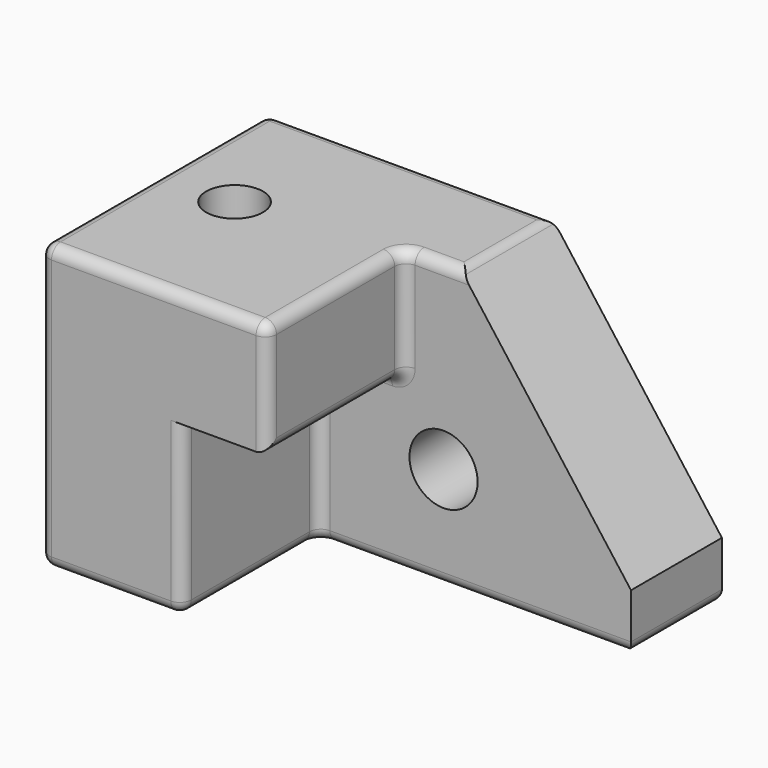
from build123d import *

# Parameters (mm, degrees)
F0_W     = 203.2
F0_H     = 127
F1_DEPTH = 127
F3_DEPTH = 76.2
F4_SIZE2 = 101.6
F4_SIZE  = 76.2
F5_R     = 5.08
F6_R     = 15.24
F7_DEPTH = 50.8
F8_R     = 12.7
F9_DEPTH = 127


with BuildPart() as f1:
    # F0 (on Front) → F1 (new body)
    with BuildSketch(Plane.XZ):
        Rectangle(F0_W, F0_H)
    extrude(amount=F1_DEPTH)

    # F2 (on face) → F3 (cut)
    with BuildSketch(Plane.XZ.offset(127)):
        Polygon((101.6, 63.5), (0, 63.5), (0, 12.7), (-38.1, 12.7), (-38.1, -63.5), (101.6, -63.5), align=None)
    extrude(amount=-F3_DEPTH, mode=Mode.SUBTRACT)

    # F4
    f4_edges = [f1.edges().sort_by_distance(p)[0] for p in [
        (101.6, -25.4, 63.5),
    ]]
    f4_side = f1.faces().sort_by_distance((-21.771429, -52.614286, 63.5))[0]
    chamfer(f4_edges, length=F4_SIZE, length2=F4_SIZE2, reference=f4_side)

    # F5
    f5_edges = [f1.edges().sort_by_distance(p)[0] for p in [
        (0, -88.9, 63.5),
        (12.7, -50.8, 63.5),
        (25.4, -25.4, 63.5),
        (-38.1, 0, 63.5),
        (-101.6, -63.5, 63.5),
        (-50.8, -127, 63.5),
        (0, -127, 38.1),
        (0, -88.9, 12.7),
        (0, -50.8, 38.1),
        (-38.1, -50.8, -25.4),
        (-38.1, -127, -25.4),
        (-38.1, -88.9, -63.5),
        (-69.85, -127, -63.5),
        (-101.6, -127, 0),
        (31.75, -50.8, -63.5),
        (101.6, -25.4, -63.5),
        (-101.6, -63.5, -63.5),
        (-101.6, 0, 0),
        (0, 0, -63.5),
        (-19.05, -50.8, 12.7),
    ]]
    fillet(f5_edges, radius=F5_R)

    # F6 (on face) → F7 (cut, through all)
    with BuildSketch(Plane.XZ.offset(50.8)):
        with Locations((17.78, -17.78)):
            Circle(F6_R)
    extrude(amount=-F7_DEPTH, mode=Mode.SUBTRACT)

    # F8 (on face) → F9 (cut, through all)
    with BuildSketch(Plane.XY.offset(63.5)):
        with Locations((-67.9840967059, -60.368321836)):
            Circle(F8_R)
    extrude(amount=-F9_DEPTH, mode=Mode.SUBTRACT)


solid = f1.part
